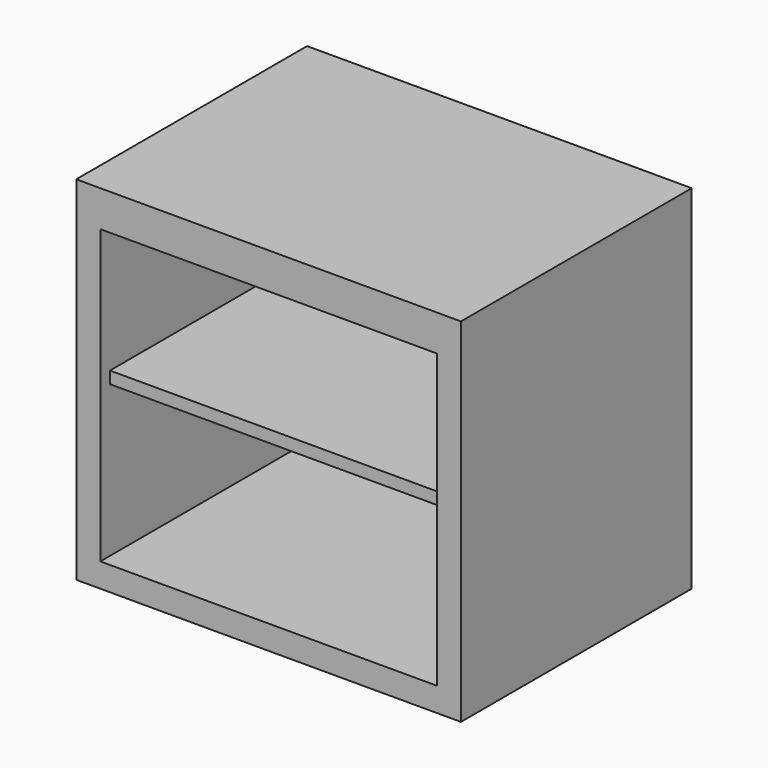
from build123d import *

# Parameters (mm, degrees)
F0_W     = 457.2
F0_H     = 558.8
F1_DEPTH = 609.6
F2_W     = 533.4
F2_H     = 463.55
F3_DEPTH = 444.5
F4_W     = 533.4
F4_H     = 19.05
F5_DEPTH = 425.45


# Not quite as in the source:
# - a feature names something its author has since deleted; it is built from what else it names


with BuildPart() as f1:
    # F0 (on Right) → F1 (new body)
    with BuildSketch(Plane.YZ):
        with Locations((-228.6, 279.4)):
            Rectangle(F0_W, F0_H)
    extrude(amount=F1_DEPTH)

    # F2 (on face) → F3 (cut)
    with BuildSketch(Plane.XZ.offset(457.2)):
        with Locations((304.8, 269.875)):
            Rectangle(F2_W, F2_H)
    extrude(amount=-F3_DEPTH, mode=Mode.SUBTRACT)

    # F4 (on face) → F5 (join)
    with BuildSketch(Plane.XZ.offset(12.7)):
        with Locations((304.8, 287.1150959969)):
            Rectangle(F4_W, F4_H)
    extrude(amount=F5_DEPTH)


solid = f1.part
